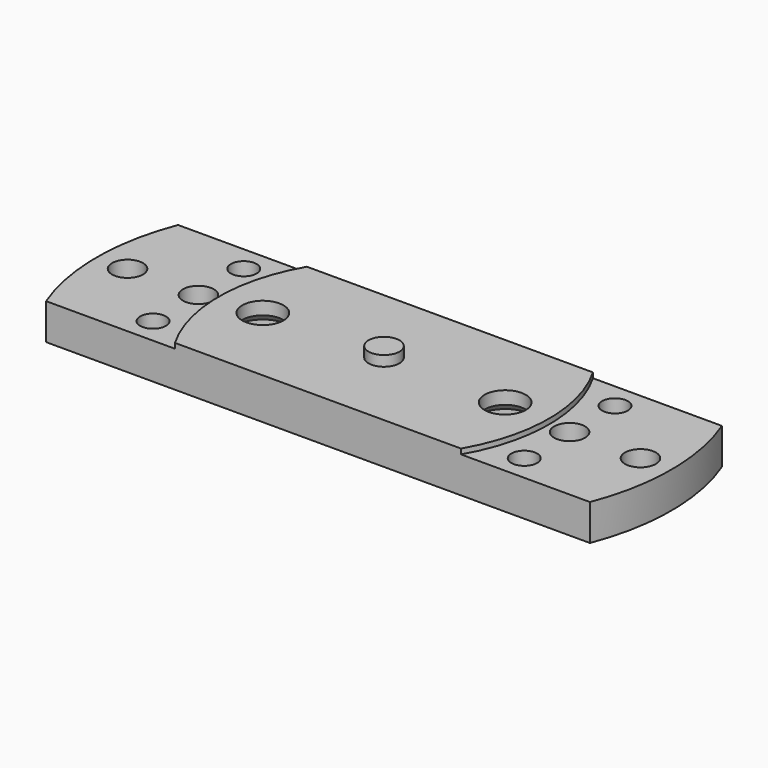
from build123d import *

# Parameters (mm, degrees)
F1_DEPTH     = 31.75
F2_W         = 377.4263709784
F2_H         = 129.2024739087
F2_R         = 9.525
F3_DEPTH     = 6.35
F4_W         = 382.6104104519
F4_H         = 158.9530184865
F5_DEPTH     = 3.175
F6_R         = 12.7
F6_R_2       = 9.525
F6_R_3       = 7.9375
F7_DEPTH     = 25.4
F8_R         = 17.4625
F9_DEPTH     = 12.7
F10_S5_R     = 17.4625
F10_T6_DEPTH = 26
F11_SIZE     = 4.76249


# Not quite as in the source:
# - a fillet or chamfer that OpenCascade refuses, or shapes differently, is made with other operations: its cross-section is extruded or revolved along the edge and cut away or added
# - a fillet or chamfer is up to 0.001 mm smaller than in the source, because OpenCascade refuses the exact size


with BuildPart() as f1:
    # F0 (on Top) → F1 (new body)
    with BuildSketch(Plane.XY):
        with BuildLine():
            Line((167.4749, 50.8), (-167.4749, 50.8))
            ThreePointArc((-167.4749, 50.8), (-176.9999, 0), (-167.4749, -50.8))
            Line((-167.4749, -50.8), (167.4749, -50.8))
            ThreePointArc((167.4749, -50.8), (176.9999, 0), (167.4749, 50.8))
        make_face()
    extrude(amount=F1_DEPTH)

    # F2 (on face) → F3 (cut)
    with BuildSketch(Plane.XY.offset(31.75)):
        with Locations((2.5683268905, -4.8314835876)):
            Rectangle(F2_W, F2_H)
        Circle(F2_R, mode=Mode.SUBTRACT)
    extrude(amount=-F3_DEPTH, mode=Mode.SUBTRACT)

    # F4 (on face) → F5 (cut)
    with BuildSketch(Plane.XY.offset(25.4)):
        with Locations((2.3195892572, -0.8801557124)):
            Rectangle(F4_W, F4_H)
        with BuildLine():
            Line((-167.4749, 50.8), (-88.1336606718, 50.8))
            Line((-88.1336606718, 50.8), (88.0661393282, 50.8))
            Line((88.0661393282, 50.8), (167.4749, 50.8))
            ThreePointArc((167.4749, 50.8), (176.9999, 0), (167.4749, -50.8))
            Line((167.4749, -50.8), (88.0661393282, -50.8))
            Line((88.0661393282, -50.8), (-88.1336606718, -50.8))
            Line((-88.1336606718, -50.8), (-167.4749, -50.8))
            ThreePointArc((-167.4749, -50.8), (-176.9999, 0), (-167.4749, 50.8))
        make_face(mode=Mode.SUBTRACT)
        with BuildLine():
            Line((167.4749, 50.8), (88.0661393282, 50.8))
            ThreePointArc((88.0661393282, 50.8), (101.6675213437, 0), (88.0661393282, -50.8))
            Line((88.0661393282, -50.8), (167.4749, -50.8))
            ThreePointArc((167.4749, -50.8), (176.9999, 0), (167.4749, 50.8))
        make_face()
        with BuildLine():
            ThreePointArc((-88.1336606718, -50.8), (-101.7350426874, 0), (-88.1336606718, 50.8))
            Line((-88.1336606718, 50.8), (-167.4749, 50.8))
            ThreePointArc((-167.4749, 50.8), (-176.9999, 0), (-167.4749, -50.8))
            Line((-167.4749, -50.8), (-88.1336606718, -50.8))
        make_face()
    extrude(amount=-F5_DEPTH, mode=Mode.SUBTRACT)

    # F6 (on face) → F7 (cut)
    with BuildSketch(Plane.XY.offset(25.4)):
        with Locations((-74.6125, 0)):
            Circle(F6_R)
        with Locations((74.6125, 0)):
            Circle(F6_R)
        with Locations((114.3, 0)):
            Circle(F6_R_2)
        with Locations((157.9499, 0)):
            Circle(F6_R_2)
        with Locations((-114.3, 0)):
            Circle(F6_R_2)
        with Locations((-157.9499, 0)):
            Circle(F6_R_2)
        with Locations((-114.3, 34.925)):
            Circle(F6_R_3)
        with Locations((-114.3, -34.925)):
            Circle(F6_R_3)
        with Locations((114.3, 34.925)):
            Circle(F6_R_3)
        with Locations((114.3, -34.925)):
            Circle(F6_R_3)
    extrude(amount=-F7_DEPTH, mode=Mode.SUBTRACT)

    # F8 (on face) → F9 (cut)
    with BuildSketch(Plane(origin=(0, 0, 0), x_dir=(1, 0, 0), z_dir=(0, 0, -1))):
        with Locations((-74.6125, 0)):
            Circle(F8_R)
        with Locations((74.6125, 0)):
            Circle(F8_R)
    extrude(amount=-F9_DEPTH, mode=Mode.SUBTRACT)

    # F10: chamfer of 4.7752 on 1 edges, made by hand


with BuildPart() as f10_tool2:
    # F10_s3 → F10_t4 (revolve)
    with BuildSketch(Plane.XZ):
        Polygon((87.3125, 17.4752), (92.0877, 12.7), (87.3125, 12.7), align=None)
    revolve(axis=Axis((74.6125, 0, 12.7), (0, 0, 1)))

    # F10_s5 → F10_t6 (intersect, symmetric)
    with BuildSketch(Plane.XY.offset(15.1)):
        with Locations((74.6125, 0)):
            Circle(F10_S5_R)
    extrude(amount=F10_T6_DEPTH, both=True, mode=Mode.INTERSECT)


with BuildPart() as f1_1:
    add(f1.part)

    # F10_t1: cut F10_tool2
    add(f10_tool2.part, mode=Mode.SUBTRACT)

    # F11 (size 4.7625 in the source; OpenCascade refuses exactly that, so slightly less here)
    f11_edges = [f1_1.edges().sort_by_distance(p)[0] for p in [
        (-87.3125, 0, 12.7),
    ]]
    chamfer(f11_edges, length=F11_SIZE)


solid = f1_1.part
